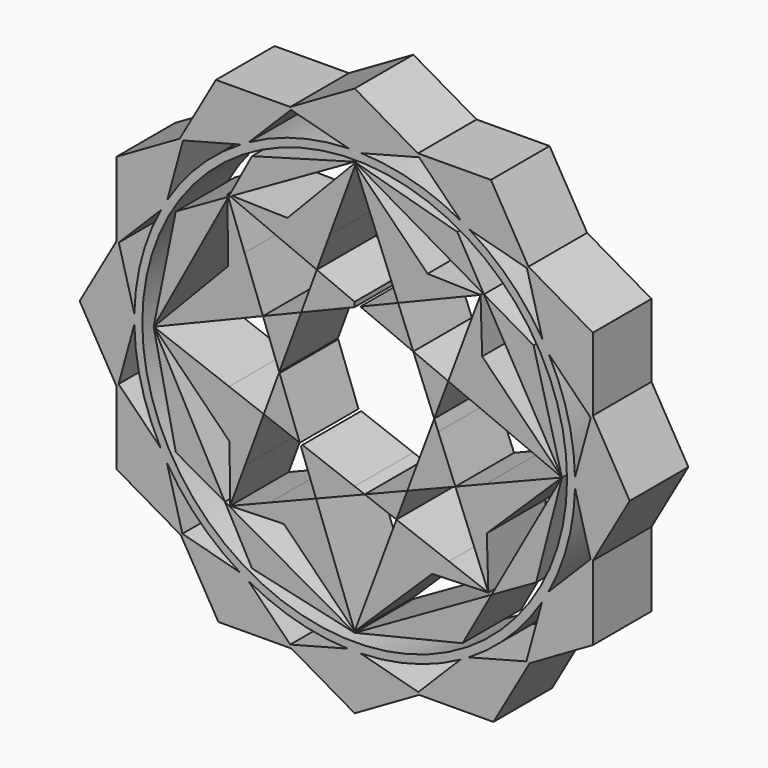
from build123d import *

# Parameters (mm, degrees)
F1_DEPTH = 15
F2_R     = 45.0945216309
F2_R_2   = 43.4508051994
F3_DEPTH = 15
F5_DEPTH = 15
F7_DEPTH = 15


with BuildPart() as f1:
    # F0 (on Front) → F1 (new body)
    with BuildSketch(Plane.XZ):
        Polygon((-48.7309247255, -13.1952988547), (-48.7309247255, -28.1348125081), (-35.5542679214, -35.742358861), align=None)
        Polygon((-56.2688417692, -0.2968929516), (-48.7309247255, -13.1952988547), (-48.7309247255, 12.9197198024), align=None)
        Polygon((-48.7309247255, 12.9197198024), (-48.7309247255, -13.1952988547), (-35.5542679214, -35.742358861), (-12.937998344, -48.7998681896), (13.1766568041, -48.6620786634), (35.7929263815, -35.6045693349), (48.7309247255, -12.9197198024), (48.7309247255, 13.1952988547), (35.5542679214, 35.742358861), (12.937998344, 48.7998681896), (-13.1766568041, 48.6620786634), (-35.7929263815, 35.6045693349), align=None)
        Polygon((-22.4719688563, -38.7747612877), (-35.2396506168, -35.3810573271), (-38.7727271377, -22.3002613209), (-48.3027714309, -12.6686410194), (-44.815912729, 0.0739152588), (-48.2607197665, 12.8279039911), (-38.6989563837, 22.4280360148), (-35.1227506697, 35.4971066226), (-22.3439438727, 38.8486765465), (-13.0210691496, 48.2089613182), (0.073770754, 44.7282973357), (13.1800207612, 48.165747642), (22.4719688563, 38.7747612877), (35.2396506168, 35.3810573271), (38.7727271377, 22.3002613209), (48.3027714309, 12.6686410194), (44.815912729, -0.0739152588), (48.2607197665, -12.8279039911), (38.6989563837, -22.4280360148), (35.1227506697, -35.4971066226), (22.3439438727, -38.8486765465), (13.0210691496, -48.2089613182), (-0.073770754, -44.7282973357), (-13.1800207612, -48.165747642), align=None, mode=Mode.SUBTRACT)
        Polygon((-12.937998344, -48.7998681896), (-35.5542679214, -35.742358861), (-27.8773040464, -48.8786928895), align=None)
        Polygon((-48.7309247255, 28.1348125081), (-48.7309247255, 12.9197198024), (-35.7929263815, 35.6045693349), align=None)
        Polygon((13.1766568041, -48.6620786634), (-12.937998344, -48.7998681896), (0, -56.2696250163), align=None)
        Polygon((-28.3915377229, 48.5817999379), (-35.7929263815, 35.6045693349), (-13.1766568041, 48.6620786634), align=None)
        Polygon((35.7929263815, -35.6045693349), (13.1766568041, -48.6620786634), (28.3915377229, -48.5817999379), align=None)
        Polygon((0, 56.2696250163), (-13.1766568041, 48.6620786634), (12.937998344, 48.7998681896), align=None)
        Polygon((48.7309247255, -12.9197198024), (35.7929263815, -35.6045693349), (48.7309247255, -28.1348125081), align=None)
        Polygon((27.8773040464, 48.8786928895), (12.937998344, 48.7998681896), (35.5542679214, 35.742358861), align=None)
        Polygon((48.7309247255, 13.1952988547), (48.7309247255, -12.9197198024), (56.2688417692, 0.2968929516), align=None)
        Polygon((48.7309247255, 28.1348125081), (35.5542679214, 35.742358861), (48.7309247255, 13.1952988547), align=None)
    extrude(amount=F1_DEPTH)

    # F2 (on Front) → F3 (join)
    with BuildSketch(Plane.XZ):
        Circle(F2_R)
        Circle(F2_R_2, mode=Mode.SUBTRACT)
    extrude(amount=F3_DEPTH)


with BuildPart() as f5:
    # F4 (on Front) → F5 (new body)
    with BuildSketch(Plane.XZ):
        Polygon((21.0088100284, 37.2609086335), (0, 43.0746637285), (26.4435683172, 27.8004036568), align=None)
    extrude(amount=F5_DEPTH)


with BuildPart() as f5b:
    # F4 (on Front) → F5, piece 2 (new body)
    with BuildSketch(Plane.XZ):
        Polygon((36.6002544761, 21.9337269664), (26.4435683172, 27.8004036568), (42.4140132964, 0), align=None)
    extrude(amount=F5_DEPTH)


with BuildPart() as f5c:
    # F4 (on Front) → F5, piece 3 (new body)
    with BuildSketch(Plane.XZ):
        Polygon((37.1287763119, -20.6124167889), (42.4140132964, 0), (28.016454869, -25.8034154438), align=None)
    extrude(amount=F5_DEPTH)


with BuildPart() as f5d:
    # F4 (on Front) → F5, piece 4 (new body)
    with BuildSketch(Plane.XZ):
        Polygon((22.0658574253, -36.4681221545), (28.016454869, -25.8034154438), (0, -41.7634954795), align=None)
    extrude(amount=F5_DEPTH)


with BuildPart() as f5e:
    # F4 (on Front) → F5, piece 5 (new body)
    with BuildSketch(Plane.XZ):
        Polygon((-21.0088100284, -36.9966439903), (0, -41.7634954795), (-26.5505858084, -26.803463658), align=None)
    extrude(amount=F5_DEPTH)


with BuildPart() as f5f:
    # F4 (on Front) → F5, piece 6 (new body)
    with BuildSketch(Plane.XZ):
        Polygon((-26.5505858084, -26.803463658), (-41.1229548705, 0), (-36.6002507508, -21.1409404874), align=None)
    extrude(amount=F5_DEPTH)


with BuildPart() as f5g:
    # F4 (on Front) → F5, piece 7 (new body)
    with BuildSketch(Plane.XZ):
        Polygon((-25.8063389802, 28.3736161663), (0, 43.0746637285), (-21.0088100284, 37.2609086335), align=None)
    extrude(amount=F5_DEPTH)


with BuildPart() as f5h:
    # F4 (on Front) → F5, piece 8 (new body)
    with BuildSketch(Plane.XZ):
        Polygon((-36.6002507508, 22.2246691792), (-41.1229548705, 0), (-25.8063389802, 28.3736161663), align=None)
    extrude(amount=F5_DEPTH)


with BuildPart() as f7:
    # F6 (on Front) → F7 (new body)
    with BuildSketch(Plane.XZ):
        Polygon((26.3766155424, 6.7493290849), (42.4140132964, 0), (26.0837073063, 16.4829244658), align=None)
        Polygon((26.3766155424, 6.7493290849), (26.0837073063, 16.4829244658), (22.8614601809, 19.7352858123), (19.1483465289, 9.7913417003), align=None)
        Polygon((22.8614601809, 19.7352858123), (26.0837073063, 16.4829244658), (25.7528220657, 27.4785287302), align=None)
    extrude(amount=F7_DEPTH)


with BuildPart() as f7b:
    # F6 (on Front) → F7, piece 2 (new body)
    with BuildSketch(Plane.XZ):
        Polygon((27.0324943927, -15.0460954219), (42.4140132964, 0), (26.768296166, -6.2665586187), align=None)
        Polygon((27.3510925472, -25.6333891302), (27.0324943927, -15.0460954219), (24.2197594366, -17.7974933047), align=None)
        Polygon((24.2197594366, -17.7974933047), (27.0324943927, -15.0460954219), (26.768296166, -6.2665586187), (20.5992374077, -8.7374436545), align=None)
    extrude(amount=F7_DEPTH)


with BuildPart() as f7c:
    # F6 (on Front) → F7, piece 3 (new body)
    with BuildSketch(Plane.XZ):
        Polygon((20.5992374077, -8.7374436545), (17.107633228, 0), (15.4922153068, 0), (11.4761063732, -10.7553838976), (12.6991779557, -11.901644134), align=None)
        Polygon((15.4922153068, 0), (17.107633228, 0), (16.2725386649, 2.0897533956), align=None)
        Polygon((10.7577255026, -12.6792515458), (12.6991779557, -11.901644134), (11.4761063732, -10.7553838976), align=None)
    extrude(amount=F7_DEPTH)


with BuildPart() as f7d:
    # F6 (on Front) → F7, piece 4 (new body)
    with BuildSketch(Plane.XZ):
        Polygon((18.2468584498, 24.3930143215), (25.7528220657, 27.4785287302), (14.9149567272, 27.7560550663), align=None)
        Polygon((5.9239221834, 27.9862894157), (14.9149567272, 27.7560550663), (0, 42.8104028106), (0.1194230796, 42.5115566712), align=None)
        Polygon((18.2468584498, 24.3930143215), (14.9149567272, 27.7560550663), (5.9239221834, 27.9862894157), (8.8959336893, 20.5490824081), align=None)
        Polygon((0.1194230796, 42.5115566712), (0, 42.8104028106), (0, 42.1864764856), align=None)
        Polygon((0, 42.1864764856), (0, 42.8104028106), (-13.7458437842, 28.4899751426), (-5.1128272098, 28.2689085963), align=None)
        Polygon((-5.1128272098, 28.2689085963), (-13.7458437842, 28.4899751426), (-17.0652528356, 25.0318129542), (-7.7432536175, 21.1086552564), align=None)
        Polygon((-17.0652528356, 25.0318129542), (-13.7458437842, 28.4899751426), (-26.029786095, 28.8045313209), align=None)
    extrude(amount=F7_DEPTH)


with BuildPart() as f7e:
    # F6 (on Front) → F7, piece 5 (new body)
    with BuildSketch(Plane.XZ):
        Polygon((15.8615745693, -25.9734119415), (27.3510925472, -25.6333891302), (19.2939769922, -22.615859628), align=None)
        Polygon((5.681125902, -26.2746939259), (15.8615745693, -25.9734119415), (19.2939769922, -22.615859628), (8.5498757596, -18.5920073916), align=None)
        Polygon((0, -41.4890944958), (15.8615745693, -25.9734119415), (5.681125902, -26.2746939259), align=None)
    extrude(amount=F7_DEPTH)


with BuildPart() as f7f:
    # F6 (on Front) → F7, piece 6 (new body)
    with BuildSketch(Plane.XZ):
        Polygon((16.2725386649, 2.0897533956), (19.1483465289, 9.7913417003), (11.9970389011, 12.8009651634), (11.9936389633, 12.7973373945), align=None)
    extrude(amount=F7_DEPTH)


with BuildPart() as f7g:
    # F6 (on Front) → F7, piece 7 (new body)
    with BuildSketch(Plane.XZ):
        Polygon((11.9912087589, 12.8034187751), (8.8959336893, 20.5490824081), (1.1512171726, 17.3654226373), align=None)
    extrude(amount=F7_DEPTH)


with BuildPart() as f7h:
    # F6 (on Front) → F7, piece 8 (new body)
    with BuildSketch(Plane.XZ):
        Polygon((-14.4781441457, -26.8712909013), (0, -41.4890944958), (-5.5112503313, -26.6059230722), align=None)
        Polygon((-25.4891159195, -27.1971515323), (-14.4781441457, -26.8712909013), (-17.3744866065, -23.9470096669), align=None)
        Polygon((-17.3744866065, -23.9470096669), (-14.4781441457, -26.8712909013), (-5.5112503313, -26.6059230722), (-7.9009291598, -20.1525780935), align=None)
    extrude(amount=F7_DEPTH)


with BuildPart() as f7i:
    # F6 (on Front) → F7, piece 9 (new body)
    with BuildSketch(Plane.XZ):
        Polygon((2.0619402633, -16.1621630342), (8.5498757596, -18.5920073916), (10.7577255026, -12.6792515458), align=None)
    extrude(amount=F7_DEPTH)


with BuildPart() as f7j:
    # F6 (on Front) → F7, piece 10 (new body)
    with BuildSketch(Plane.XZ):
        Polygon((-11.2206694735, -11.1875953401), (-15.363445013, 0), (-15.4978345771, 0), (-18.5933925786, -8.4263826791), align=None)
    extrude(amount=F7_DEPTH)


with BuildPart() as f7k:
    # F6 (on Front) → F7, piece 11 (new body)
    with BuildSketch(Plane.XZ):
        Polygon((-10.9451077096, 12.392925217), (0, 16.8921859744), (0, 17.8499116838), (-7.7432536175, 21.1086552564), align=None)
    extrude(amount=F7_DEPTH)


with BuildPart() as f7l:
    # F6 (on Front) → F7, piece 12 (new body)
    with BuildSketch(Plane.XZ):
        Polygon((2.0619402633, -16.1621630342), (0, -15.3899306473), (0, -16.988029271), align=None)
        Polygon((0, -16.988029271), (0, -15.3899306473), (-10.6761252657, -11.3915365894), (-11.0123159489, -11.7502555416), (-7.9009291598, -20.1525780935), align=None)
    extrude(amount=F7_DEPTH)


with BuildPart() as f7m:
    # F6 (on Front) → F7, piece 13 (new body)
    with BuildSketch(Plane.XZ):
        Polygon((-15.4309072213, 0.182182182), (-11.018522331, 12.1930841242), (-11.1303132584, 12.3167918358), (-18.7625699469, 9.1793614951), align=None)
    extrude(amount=F7_DEPTH)


with BuildPart() as f7n:
    # F6 (on Front) → F7, piece 14 (new body)
    with BuildSketch(Plane.XZ):
        Polygon((-22.5260726641, 19.3427278322), (-26.029786095, 28.8045313209), (-25.9044566656, 15.8231255082), align=None)
        Polygon((-25.8123355426, 6.2813787128), (-18.7625699469, 9.1793614951), (-22.5260726641, 19.3427278322), (-25.9044566656, 15.8231255082), align=None)
        Polygon((-25.8123355426, 6.2813787128), (-25.9044566656, 15.8231255082), (-41.0927049816, 0), align=None)
    extrude(amount=F7_DEPTH)


with BuildPart() as f7o:
    # F6 (on Front) → F7, piece 15 (new body)
    with BuildSketch(Plane.XZ):
        Polygon((-25.6006807042, -15.6414638428), (-25.4891159195, -27.1971515323), (-22.422701042, -18.8500990147), align=None)
        Polygon((-22.422701042, -18.8500990147), (-18.5933925786, -8.4263826791), (-25.6960205691, -5.7663253225), (-25.6006807042, -15.6414638428), align=None)
        Polygon((-41.0927049816, 0), (-25.6006807042, -15.6414638428), (-25.6960205691, -5.7663253225), align=None)
    extrude(amount=F7_DEPTH)


solid = Compound([f1.part, f5.part, f5b.part, f5c.part, f5d.part, f5e.part, f5f.part, f5g.part, f5h.part, f7.part, f7b.part, f7c.part, f7d.part, f7e.part, f7f.part, f7g.part, f7h.part, f7i.part, f7j.part, f7k.part, f7l.part, f7m.part, f7n.part, f7o.part])
